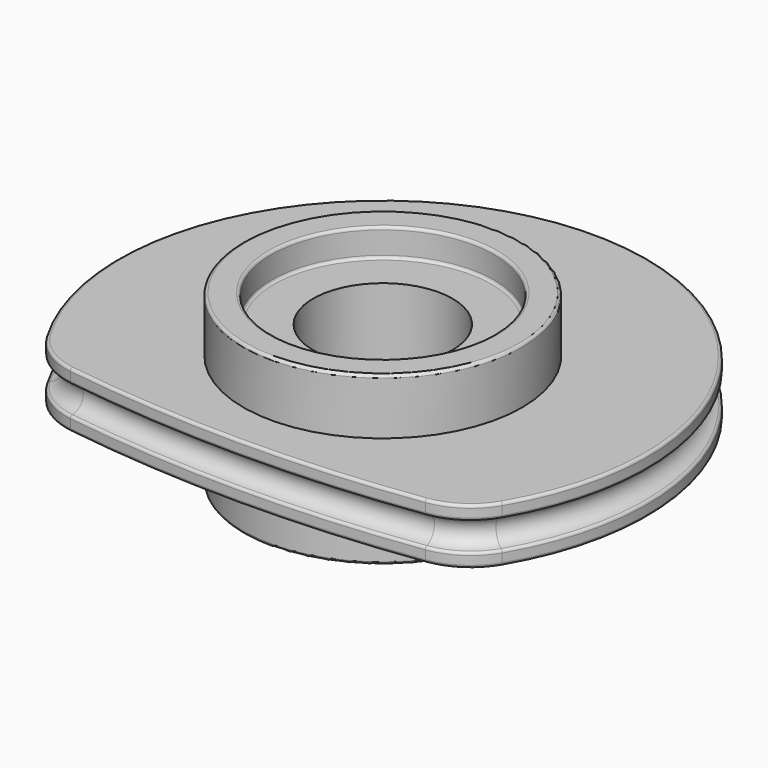
from build123d import *

# Parameters (mm, degrees)
F3_R           = 5
F4_DEPTH       = 3
F4_DEPTH_BACK  = 3
F6_R           = 10
F6_R_2         = 2.5
F7_DEPTH       = 1
F7_DEPTH_BACK  = 1
F10_R          = 2.5
F11_DEPTH      = 3.001
F11_DEPTH_BACK = 3.001
F12_R          = 4
F13_DEPTH      = 1
F14_R          = 0.1


# Not quite as in the source:
# - a feature names something its author has since deleted; it is built from what else it names


with BuildPart() as f4:
    # F3 (on Top) → F4 (new body, two sides)
    with BuildSketch(Plane.XY) as f4_sk:
        Circle(F3_R)
    extrude(amount=F4_DEPTH)
    extrude(f4_sk.sketch, amount=-F4_DEPTH_BACK)

    # F6 (on Top) → F7 (join, two sides)
    with BuildSketch(Plane.XY) as f7_sk:
        Circle(F6_R)
        Circle(F6_R_2, mode=Mode.SUBTRACT)
    extrude(amount=F7_DEPTH)
    extrude(f7_sk.sketch, amount=-F7_DEPTH_BACK)

    # F9: sweep along a path in F5
    with BuildLine(Plane.XY) as f9_path:
        ThreePointArc((7.7362851991, -4.5989010989), (0, 9), (-7.7362851991, -4.5989010989))
        ThreePointArc((-7.7362851991, -4.5989010989), (-7.1255538214, -5.2416614557), (-6.2969763249, -5.5572450805))
        ThreePointArc((-6.2969763249, -5.5572450805), (0, -6), (6.2969763249, -5.5572450805))
        ThreePointArc((6.2969763249, -5.5572450805), (7.1255538214, -5.2416614557), (7.7362851991, -4.5989010989))
    # F8 (on Front) → F9 (sweep, cut)
    with BuildSketch(Plane.XZ):
        with BuildLine():
            ThreePointArc((9.5, 0.5916079783), (9.4763762616, 0.5270582559), (9.4166666667, 0.4930066486))
            ThreePointArc((9.4166666667, 0.4930066486), (9, 0), (9.4166666667, -0.4930066486))
            ThreePointArc((9.4166666667, -0.4930066486), (9.4763762616, -0.5270582559), (9.5, -0.5916079783))
            Line((9.5, -0.5916079783), (9.5, -0.9))
            ThreePointArc((9.5, -0.9), (9.4707106781, -0.9707106781), (9.4, -1))
            Line((9.4, -1), (8.5, -1))
            Line((8.5, -1), (8.5, -2))
            Line((8.5, -2), (18, -2))
            Line((18, -2), (18, 2))
            Line((18, 2), (8.5, 2))
            Line((8.5, 2), (8.5, 1))
            Line((8.5, 1), (9.4, 1))
            ThreePointArc((9.4, 1), (9.4707106781, 0.9707106781), (9.5, 0.9))
            Line((9.5, 0.9), (9.5, 0.5916079783))
        make_face()
    sweep(path=f9_path.line, mode=Mode.SUBTRACT)

    # F10 (on Top) → F11 (cut, two sides)
    with BuildSketch(Plane.XY) as f11_sk:
        Circle(F10_R)
    extrude(amount=-F11_DEPTH, mode=Mode.SUBTRACT)
    extrude(f11_sk.sketch, amount=F11_DEPTH_BACK, mode=Mode.SUBTRACT)

    # F12 (on face) → F13 (cut)
    with BuildSketch(Plane.XY.offset(3)):
        Circle(F12_R)
    extrude(amount=-F13_DEPTH, mode=Mode.SUBTRACT)

    # F14
    f14_edges = [f4.edges().sort_by_distance(p)[0] for p in [
        (-4, 0, 3),
        (-4, 0, 2),
        (-5, 0, 3),
        (-5, 0, -1),
        (-5, 0, -3),
    ]]
    fillet(f14_edges, radius=F14_R)


solid = f4.part
